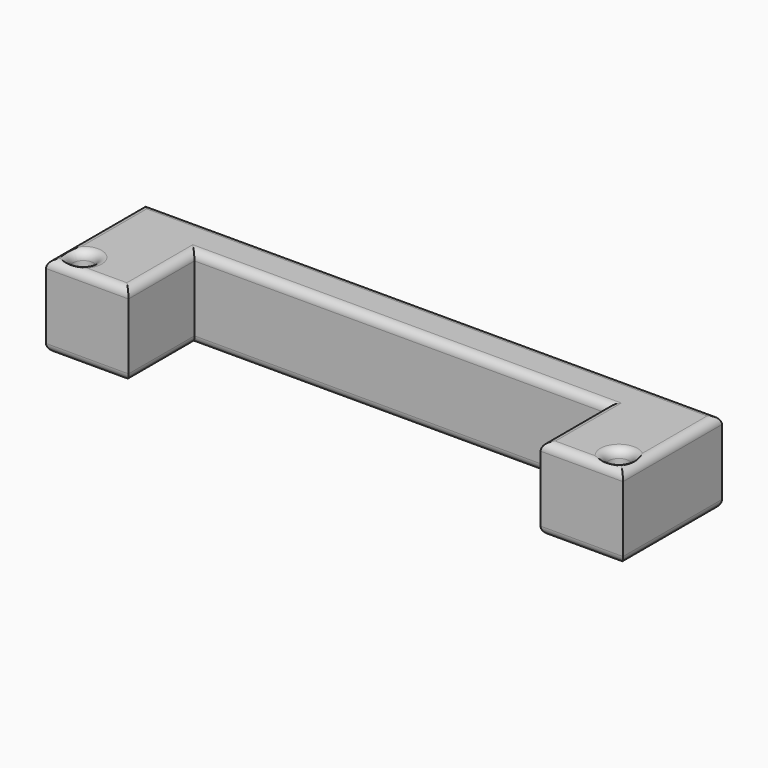
from build123d import *

# Parameters (mm, degrees)
F1_DEPTH     = 20
F3_D         = 5
F5_T1_DEPTH  = 150
F5_T3_DEPTH  = 40
F5_T5_DEPTH  = 30
F5_T7_DEPTH  = 25
F5_T9_DEPTH  = 100
F5_T11_DEPTH = 30
F5_T25_DEPTH = 30
F5_T29_DEPTH = 105
F5_T36_DEPTH = 105
F5_T40_DEPTH = 30
F5_T47_DEPTH = 105
F5_T51_DEPTH = 30
F5_T58_DEPTH = 30
F5_T62_DEPTH = 105


# Not quite as in the source:
# - a fillet or chamfer that OpenCascade refuses, or shapes differently, is made with other operations: its cross-section is extruded or revolved along the edge and cut away or added


with BuildPart() as f1:
    # F0 (on Top) → F1 (new body)
    with BuildSketch(Plane.XY):
        Polygon((70, 30), (0, 30), (0, 20), (50, 20), (50, 0), (70, 0), align=None)
    extrude(amount=F1_DEPTH)

    # F3 (through all)
    with Locations(Plane.XY.offset(20)):
        with Locations((65, 5)):
            Hole(F3_D / 2)

    # F4: F1 across face


with BuildPart() as f1_1:
    add(f1.part)
    add(f1.part.mirror(Plane(origin=(0, 25, 10), x_dir=(0, -1, 0), z_dir=(-1, 0, 0))))

    # F5: fillet of radius 2 on 20 edges, made by hand

    # F5_s2 → F5_t1 (cut)
    with BuildSketch(Plane.YZ.offset(-75)):
        with BuildLine():
            ThreePointArc((30, 2), (29.4142135624, 0.5857864376), (28, 0))
            Line((28, 0), (30, 0))
            Line((30, 0), (30, 2))
        make_face()
        with BuildLine():
            ThreePointArc((30, 18), (29.4142135624, 19.4142135624), (28, 20))
            Line((28, 20), (30, 20))
            Line((30, 20), (30, 18))
        make_face()
    extrude(amount=F5_T1_DEPTH, mode=Mode.SUBTRACT)

    # F5_s4 → F5_t3 (cut)
    with BuildSketch(Plane.XZ.offset(-35)):
        with BuildLine():
            ThreePointArc((-68, 0), (-69.4142135624, 0.5857864376), (-70, 2))
            Line((-70, 2), (-70, 0))
            Line((-70, 0), (-68, 0))
        make_face()
        with BuildLine():
            ThreePointArc((68, 0), (69.4142135624, 0.5857864376), (70, 2))
            Line((70, 2), (70, 0))
            Line((70, 0), (68, 0))
        make_face()
        with BuildLine():
            ThreePointArc((-70, 18), (-69.4142135624, 19.4142135624), (-68, 20))
            Line((-68, 20), (-70, 20))
            Line((-70, 20), (-70, 18))
        make_face()
        with BuildLine():
            ThreePointArc((68, 20), (69.4142135624, 19.4142135624), (70, 18))
            Line((70, 18), (70, 20))
            Line((70, 20), (68, 20))
        make_face()
    extrude(amount=F5_T3_DEPTH, mode=Mode.SUBTRACT)

    # F5_s6 → F5_t5 (cut)
    with BuildSketch(Plane.YZ.offset(-75)):
        with BuildLine():
            ThreePointArc((2, 0), (0.5857864376, 0.5857864376), (0, 2))
            Line((0, 2), (0, 0))
            Line((0, 0), (2, 0))
        make_face()
        with BuildLine():
            ThreePointArc((0, 18), (0.5857864376, 19.4142135624), (2, 20))
            Line((2, 20), (0, 20))
            Line((0, 20), (0, 18))
        make_face()
    extrude(amount=F5_T5_DEPTH, mode=Mode.SUBTRACT)

    # F5_s8 → F5_t7 (cut)
    with BuildSketch(Plane.XZ.offset(-20)):
        with BuildLine():
            ThreePointArc((-52, 0), (-50.5857864376, 0.5857864376), (-50, 2))
            Line((-50, 2), (-50, 0))
            Line((-50, 0), (-52, 0))
        make_face()
        with BuildLine():
            ThreePointArc((52, 0), (50.5857864376, 0.5857864376), (50, 2))
            Line((50, 2), (50, 0))
            Line((50, 0), (52, 0))
        make_face()
        with BuildLine():
            ThreePointArc((-50, 18), (-50.5857864376, 19.4142135624), (-52, 20))
            Line((-52, 20), (-50, 20))
            Line((-50, 20), (-50, 18))
        make_face()
        with BuildLine():
            ThreePointArc((50, 18), (50.5857864376, 19.4142135624), (52, 20))
            Line((52, 20), (50, 20))
            Line((50, 20), (50, 18))
        make_face()
    extrude(amount=F5_T7_DEPTH, mode=Mode.SUBTRACT)

    # F5_s10 → F5_t9 (cut)
    with BuildSketch(Plane.YZ.offset(-50)):
        with BuildLine():
            ThreePointArc((22, 0), (20.5857864376, 0.5857864376), (20, 2))
            Line((20, 2), (20, 0))
            Line((20, 0), (22, 0))
        make_face()
        with BuildLine():
            ThreePointArc((20, 18), (20.5857864376, 19.4142135624), (22, 20))
            Line((22, 20), (20, 20))
            Line((20, 20), (20, 18))
        make_face()
    extrude(amount=F5_T9_DEPTH, mode=Mode.SUBTRACT)

    # F5_s12 → F5_t11 (cut)
    with BuildSketch(Plane.YZ.offset(45)):
        with BuildLine():
            ThreePointArc((2, 0), (0.5857864376, 0.5857864376), (0, 2))
            Line((0, 2), (0, 0))
            Line((0, 0), (2, 0))
        make_face()
        with BuildLine():
            ThreePointArc((0, 18), (0.5857864376, 19.4142135624), (2, 20))
            Line((2, 20), (0, 20))
            Line((0, 20), (0, 18))
        make_face()
    extrude(amount=F5_T11_DEPTH, mode=Mode.SUBTRACT)

    # F5_s13 → F5_t14 (revolve, cut)
    with BuildSketch(Plane.XZ.offset(-5)):
        with BuildLine():
            ThreePointArc((69.5, 0), (68.0857864376, 0.5857864376), (67.5, 2))
            Line((67.5, 2), (67.5, 0))
            Line((67.5, 0), (69.5, 0))
        make_face()
    revolve(axis=Axis((65, 5, 0), (0, 0, 1)), mode=Mode.SUBTRACT)

    # F5_s15 → F5_t16 (revolve, cut)
    with BuildSketch(Plane.XZ.offset(-5)):
        with BuildLine():
            ThreePointArc((-69.5, 0), (-68.0857864376, 0.5857864376), (-67.5, 2))
            Line((-67.5, 2), (-67.5, 0))
            Line((-67.5, 0), (-69.5, 0))
        make_face()
    revolve(axis=Axis((-65, 5, 0), (0, 0, -1)), mode=Mode.SUBTRACT)

    # F5_s17 → F5_t18 (revolve, cut)
    with BuildSketch(Plane.XZ.offset(-5)):
        with BuildLine():
            ThreePointArc((67.5, 18), (68.0857864376, 19.4142135624), (69.5, 20))
            Line((69.5, 20), (67.5, 20))
            Line((67.5, 20), (67.5, 18))
        make_face()
    revolve(axis=Axis((65, 5, 20), (0, 0, 1)), mode=Mode.SUBTRACT)

    # F5_s19 → F5_t20 (revolve, cut)
    with BuildSketch(Plane.XZ.offset(-5)):
        with BuildLine():
            ThreePointArc((-67.5, 18), (-68.0857864376, 19.4142135624), (-69.5, 20))
            Line((-69.5, 20), (-67.5, 20))
            Line((-67.5, 20), (-67.5, 18))
        make_face()
    revolve(axis=Axis((-65, 5, 20), (0, 0, -1)), mode=Mode.SUBTRACT)


with BuildPart() as f5_tool23:
    # F5_s24 → F5_t25 (new body)
    with BuildSketch(Plane.XZ.offset(-25)):
        with BuildLine():
            ThreePointArc((-52, 0), (-50.5857864376, 0.5857864376), (-50, 2))
            Line((-50, 2), (-50, 0))
            Line((-50, 0), (-52, 0))
        make_face()
    extrude(amount=F5_T25_DEPTH)

    split(bisect_by=Plane.XZ.offset(-20), keep=Keep.BOTTOM)


with BuildPart() as f5_tool27:
    # F5_s28 → F5_t29 (new body)
    with BuildSketch(Plane.YZ.offset(50)):
        with BuildLine():
            ThreePointArc((22, 0), (20.5857864376, 0.5857864376), (20, 2))
            Line((20, 2), (20, 0))
            Line((20, 0), (22, 0))
        make_face()
    extrude(amount=-F5_T29_DEPTH)

    split(bisect_by=Plane.YZ.offset(-50), keep=Keep.BOTTOM)


with BuildPart() as f5_tool23_1:
    add(f5_tool23.part)

    # F5_t31: intersect F5_tool27
    add(f5_tool27.part, mode=Mode.INTERSECT)


with BuildPart() as f1_2:
    add(f1_1.part)

    # F5_t21: cut F5_tool23
    add(f5_tool23_1.part, mode=Mode.SUBTRACT)


with BuildPart() as f5_tool34:
    # F5_s35 → F5_t36 (new body)
    with BuildSketch(Plane.YZ.offset(55)):
        with BuildLine():
            ThreePointArc((22, 0), (20.5857864376, 0.5857864376), (20, 2))
            Line((20, 2), (20, 0))
            Line((20, 0), (22, 0))
        make_face()
    extrude(amount=-F5_T36_DEPTH)

    split(bisect_by=Plane.YZ.offset(50), keep=Keep.TOP)


with BuildPart() as f5_tool38:
    # F5_s39 → F5_t40 (new body)
    with BuildSketch(Plane.XZ.offset(-25)):
        with BuildLine():
            ThreePointArc((52, 0), (50.5857864376, 0.5857864376), (50, 2))
            Line((50, 2), (50, 0))
            Line((50, 0), (52, 0))
        make_face()
    extrude(amount=F5_T40_DEPTH)

    split(bisect_by=Plane.XZ.offset(-20), keep=Keep.BOTTOM)


with BuildPart() as f5_tool34_1:
    add(f5_tool34.part)

    # F5_t42: intersect F5_tool38
    add(f5_tool38.part, mode=Mode.INTERSECT)


with BuildPart() as f1_3:
    add(f1_2.part)

    # F5_t32: cut F5_tool34
    add(f5_tool34_1.part, mode=Mode.SUBTRACT)


with BuildPart() as f5_tool45:
    # F5_s46 → F5_t47 (new body)
    with BuildSketch(Plane.YZ.offset(-55)):
        with BuildLine():
            ThreePointArc((20, 18), (20.5857864376, 19.4142135624), (22, 20))
            Line((22, 20), (20, 20))
            Line((20, 20), (20, 18))
        make_face()
    extrude(amount=F5_T47_DEPTH)

    split(bisect_by=Plane.YZ.offset(-50), keep=Keep.BOTTOM)


with BuildPart() as f5_tool49:
    # F5_s50 → F5_t51 (new body)
    with BuildSketch(Plane.XZ.offset(-25)):
        with BuildLine():
            ThreePointArc((-50, 18), (-50.5857864376, 19.4142135624), (-52, 20))
            Line((-52, 20), (-50, 20))
            Line((-50, 20), (-50, 18))
        make_face()
    extrude(amount=F5_T51_DEPTH)

    split(bisect_by=Plane.XZ.offset(-20), keep=Keep.BOTTOM)


with BuildPart() as f5_tool45_1:
    add(f5_tool45.part)

    # F5_t53: intersect F5_tool49
    add(f5_tool49.part, mode=Mode.INTERSECT)


with BuildPart() as f1_4:
    add(f1_3.part)

    # F5_t43: cut F5_tool45
    add(f5_tool45_1.part, mode=Mode.SUBTRACT)


with BuildPart() as f5_tool56:
    # F5_s57 → F5_t58 (new body)
    with BuildSketch(Plane.XZ.offset(-25)):
        with BuildLine():
            ThreePointArc((50, 18), (50.5857864376, 19.4142135624), (52, 20))
            Line((52, 20), (50, 20))
            Line((50, 20), (50, 18))
        make_face()
    extrude(amount=F5_T58_DEPTH)

    split(bisect_by=Plane.XZ.offset(-20), keep=Keep.BOTTOM)


with BuildPart() as f5_tool60:
    # F5_s61 → F5_t62 (new body)
    with BuildSketch(Plane.YZ.offset(-50)):
        with BuildLine():
            ThreePointArc((20, 18), (20.5857864376, 19.4142135624), (22, 20))
            Line((22, 20), (20, 20))
            Line((20, 20), (20, 18))
        make_face()
    extrude(amount=F5_T62_DEPTH)

    split(bisect_by=Plane.YZ.offset(50), keep=Keep.TOP)


with BuildPart() as f5_tool56_1:
    add(f5_tool56.part)

    # F5_t64: intersect F5_tool60
    add(f5_tool60.part, mode=Mode.INTERSECT)


with BuildPart() as f1_5:
    add(f1_4.part)

    # F5_t54: cut F5_tool56
    add(f5_tool56_1.part, mode=Mode.SUBTRACT)


solid = f1_5.part
